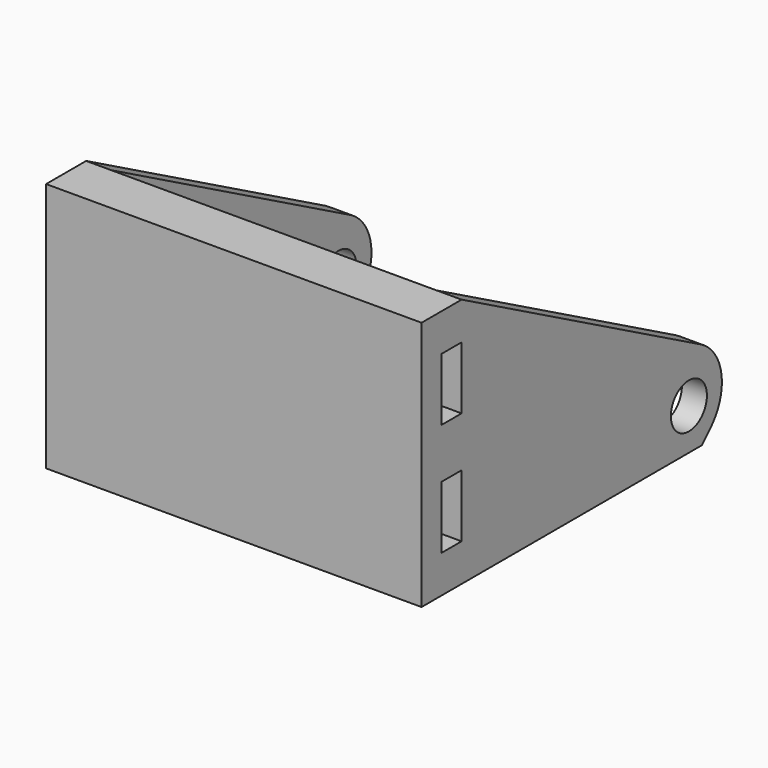
from build123d import *

# Parameters (mm, degrees)
F1_DEPTH    = 20
F2_R        = 1.8
F3_DEPTH    = 30.001
F4_SIZE2    = 14
F4_SIZE     = 26
F5_SIZE     = 2
F6_R        = 4
F7_T1_DEPTH = 13.9458816311
F7_T3_DEPTH = 13.9458816311
F8_W        = 2
F8_H        = 5
F9_DEPTH    = 30.001
F10_SIZE    = 1.99999


# Not quite as in the source:
# - a fillet or chamfer that OpenCascade refuses, or shapes differently, is made with other operations: its cross-section is extruded or revolved along the edge and cut away or added
# - a fillet or chamfer is up to 0.001 mm smaller than in the source, because OpenCascade refuses the exact size


with BuildPart() as f1:
    # F0 (on Top) → F1 (new body)
    with BuildSketch(Plane.XY):
        Polygon((15, 13), (13, 13), (13, -13), (-13, -13), (-13, 13), (-15, 13), (-15, -17), (15, -17), align=None)
    extrude(amount=F1_DEPTH)

    # F2 (on face) → F3 (cut, through all)
    with BuildSketch(Plane.YZ.offset(15)):
        with Locations((9.7, 3.3)):
            Circle(F2_R)
    extrude(amount=-F3_DEPTH, mode=Mode.SUBTRACT)

    # F4
    f4_edges = [f1.edges().sort_by_distance(p)[0] for p in [
        (14, 13, 20),
        (-14, 13, 20),
    ]]
    f4_side = f1.faces().sort_by_distance((14, 12.575736, 20))[0]
    chamfer(f4_edges, length=F4_SIZE, length2=F4_SIZE2, reference=f4_side)

    # F5
    f5_edges = [f1.edges().sort_by_distance(p)[0] for p in [
        (14, 13, 0),
        (-14, 13, 0),
    ]]
    chamfer(f5_edges, length=F5_SIZE)

    # F6
    f6_edges = [f1.edges().sort_by_distance(p)[0] for p in [
        (14, 13, 2),
        (-14, 13, 2),
    ]]
    fillet(f6_edges, radius=F6_R)

    # F7: fillet of radius 4 on 2 edges, made by hand

    # F7_s2 → F7_t1 (cut)
    with BuildSketch(Plane.YZ.offset(7.0270591844)):
        with BuildLine():
            ThreePointArc((13, 3.6108236738), (12.4340644409, 5.66197004), (10.8963992921, 7.1327080735))
            Line((10.8963992921, 7.1327080735), (13, 6))
            Line((13, 6), (13, 3.6108236738))
        make_face()
    extrude(amount=F7_T1_DEPTH, mode=Mode.SUBTRACT)

    # F7_s4 → F7_t3 (cut)
    with BuildSketch(Plane.YZ.offset(-20.9729408156)):
        with BuildLine():
            ThreePointArc((10.8963992921, 7.1327080735), (12.4340644409, 5.66197004), (13, 3.6108236738))
            Line((13, 3.6108236738), (13, 6))
            Line((13, 6), (10.8963992921, 7.1327080735))
        make_face()
    extrude(amount=F7_T3_DEPTH, mode=Mode.SUBTRACT)

    # F8 (on face) → F9 (cut, through all)
    with BuildSketch(Plane.YZ.offset(15)):
        with Locations((-14, 14.5)):
            Rectangle(F8_W, F8_H)
        with Locations((-14, 5.5)):
            Rectangle(F8_W, F8_H)
    extrude(amount=-F9_DEPTH, mode=Mode.SUBTRACT)

    # F10 (size 2 in the source; OpenCascade refuses exactly that, so slightly less here)
    f10_edges = [f1.edges().sort_by_distance(p)[0] for p in [
        (0, -13, 8),
        (0, -13, 17),
    ]]
    chamfer(f10_edges, length=F10_SIZE)


solid = f1.part
